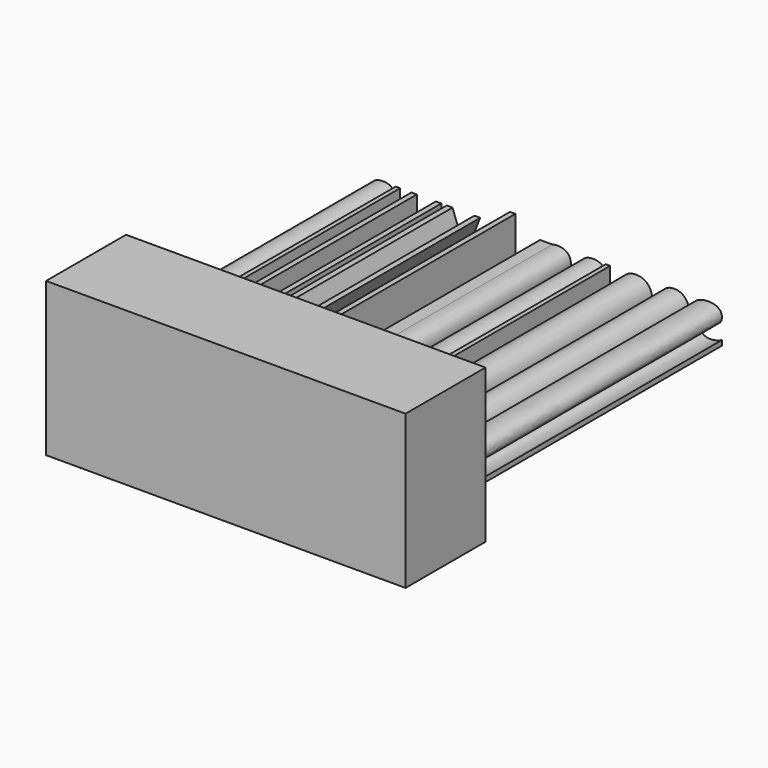
from build123d import *

# Parameters (mm, degrees)
F0_W         = 91.3478210568
F0_H         = 38.9910489321
F1_DEPTH     = 25.4
F2_TEXT_SIZE = 16.9378275224
F3_DEPTH     = 76.2


# Not quite as in the source:
# - Text() gives the source's letters only with a copy of the font that has no kerning and outlines rounded to 1/6400 em; it was checked with that copy


with BuildPart() as f1:
    # F0 (on Front) → F1 (new body)
    with BuildSketch(Plane.XZ):
        with Locations((45.6739105284, 19.495524466)):
            Rectangle(F0_W, F0_H)
    extrude(amount=F1_DEPTH)

    # F2 (on face) → F3 (join)
    with BuildSketch(Plane(origin=(0, 0, 0), x_dir=(-1, 0, 0), z_dir=(0, 1, 0))):
        with Locations((-91.3478210568, 12.1869602079)):
            Text('seong hyun', F2_TEXT_SIZE, font='Open Sans', text_align=(TextAlign.LEFT, TextAlign.BOTTOM))
    extrude(amount=F3_DEPTH)


solid = f1.part
